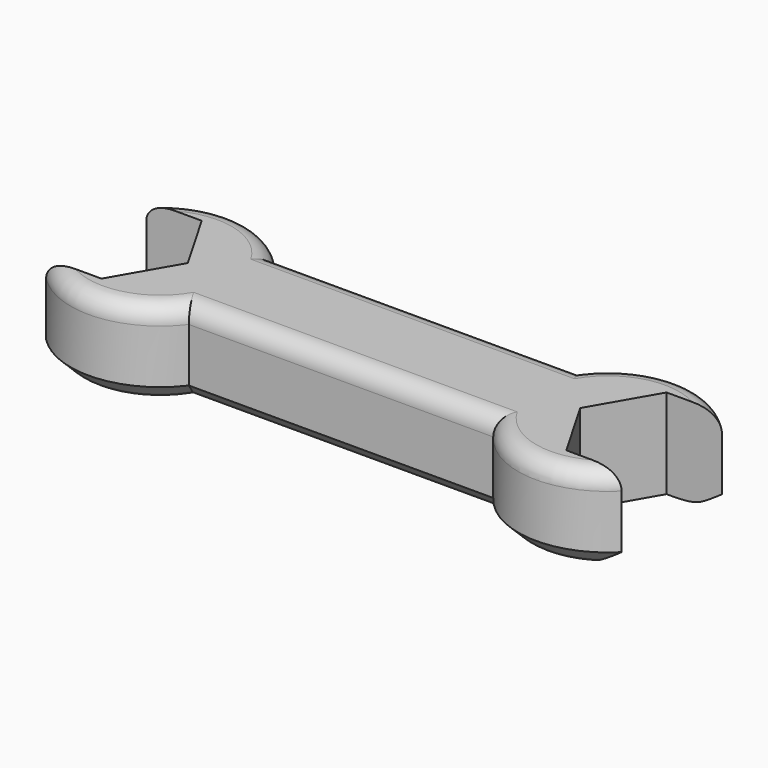
from build123d import *

# Parameters (mm, degrees)
F1_DEPTH = 6.35
F3_DEPTH = 12.701
F6_R     = 2.54
F7_SIZE  = 2.54
F8_R     = 2.54


with BuildPart() as f1:
    # F0 (on Top) → F1 (new body, symmetric)
    with BuildSketch(Plane.XY):
        with BuildLine():
            Line((21.59, 7.62), (-21.59, 7.62))
            ThreePointArc((-21.59, 7.62), (-44.45, 0), (-21.59, -7.62))
            Line((-21.59, -7.62), (21.59, -7.62))
            ThreePointArc((21.59, -7.62), (44.45, 0), (21.59, 7.62))
        make_face()
    extrude(amount=F1_DEPTH, both=True)

    # F4: F3 across plane


with BuildPart() as f3:
    # F2 (on face) → F3 (new body, through all)
    with BuildSketch(Plane.XY.offset(6.35)):
        Polygon((-27.8347122138, 0), (-32.9673561069, 8.89), (-43.2326438931, 8.89), (-48.3652877862, 0), (-43.2326438931, -8.89), (-32.9673561069, -8.89), align=None)
    extrude(amount=-F3_DEPTH)


with BuildPart() as f1_1:
    add(f1.part)
    add(f3.part.mirror(Plane.YZ), mode=Mode.SUBTRACT)

    # F5: cut F3
    add(f3.part, mode=Mode.SUBTRACT)

    # F6
    f6_edges = [f1_1.edges().sort_by_distance(p)[0] for p in [
        (0, -7.62, 6.35),
        (-30.913065, -12.672393, 6.35),
        (-30.913065, 12.672393, 6.35),
        (0, 7.62, 6.35),
        (30.913065, 12.672393, 6.35),
        (30.913065, -12.672393, 6.35),
    ]]
    fillet(f6_edges, radius=F6_R)

    # F7
    f7_edges = [f1_1.edges().sort_by_distance(p)[0] for p in [
        (-30.913065, -12.672393, -6.35),
        (0, -7.62, -6.35),
        (30.913065, -12.672393, -6.35),
        (30.913065, 12.672393, -6.35),
        (0, 7.62, -6.35),
        (-30.913065, 12.672393, -6.35),
    ]]
    chamfer(f7_edges, length=F7_SIZE)

    # F8
    f8_edges = [f1_1.edges().sort_by_distance(p)[0] for p in [
        (-29.031016, -9.789419, -6.35),
        (0, -5.08, -6.35),
        (29.031016, -9.789419, -6.35),
        (29.031016, 9.789419, -6.35),
        (0, 5.08, -6.35),
        (-29.031016, 9.789419, -6.35),
    ]]
    fillet(f8_edges, radius=F8_R)


solid = f1_1.part
